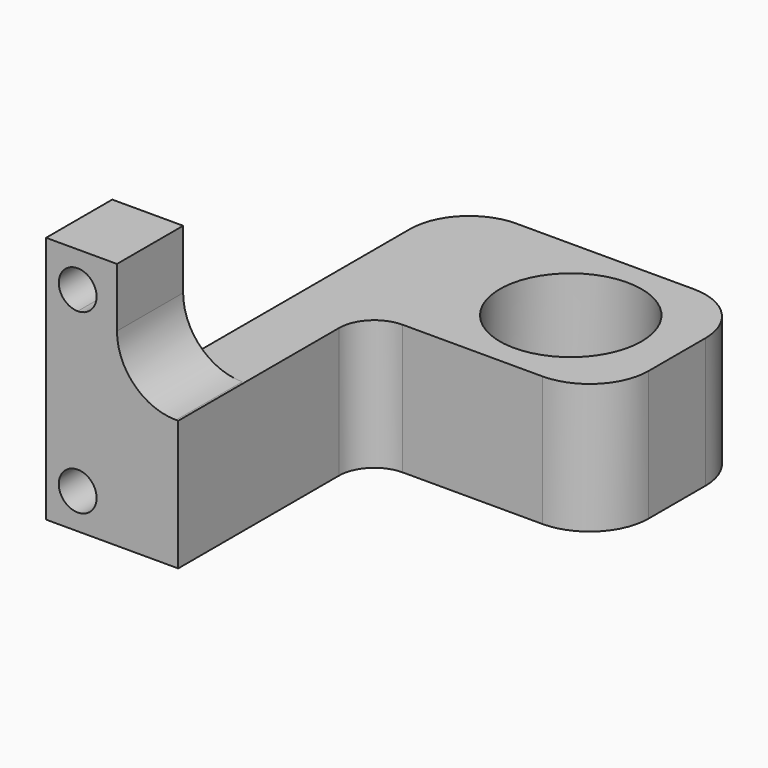
from build123d import *

# Parameters (mm, degrees)
F0_W     = 31
F0_H     = 36
F1_DEPTH = 4
F2_R     = 6
F2_W     = 6
F2_H     = 29
F2_W_2   = 19.817460835
F2_H_2   = 20
F3_DEPTH = 25
F4_W     = 6
F4_H     = 7
F4_R     = 6
F5_DEPTH = 7
F6_DEPTH = 17
F8_DEPTH = 25
F9_F1_R  = 5
F9_F2_R  = 5
F10_R    = 3


# Not quite as in the source:
# - two fillets or chamfers of one size are made in one step


with BuildPart() as f1:
    # F0 (on Top) → F1 (new body)
    with BuildSketch(Plane.XY):
        with Locations((15.5, 18)):
            Rectangle(F0_W, F0_H)
    extrude(amount=F1_DEPTH)

    # F2 (on face) → F3 (cut)
    with BuildSketch(Plane.XY.offset(4)):
        with Locations((22, 28)):
            Circle(F2_R)
        with Locations((3, 21.5)):
            Rectangle(F2_W, F2_H)
        with Locations((21.0912695825, 10)):
            Rectangle(F2_W_2, F2_H_2)
    extrude(amount=-F3_DEPTH, mode=Mode.SUBTRACT)

    # F4 (on face) → F5 (join)
    with BuildSketch(Plane.XY.offset(4)):
        with Locations((3, 3.5)):
            Rectangle(F4_W, F4_H)
        Polygon((6, 36), (6, 7), (6, 0), (11.182539165, 0), (11.182539165, 20), (31, 20), (31, 36), align=None)
        with Locations((22, 28)):
            Circle(F4_R, mode=Mode.SUBTRACT)
    extrude(amount=F5_DEPTH)

    # F4 (on face) → F6 (join)
    with BuildSketch(Plane.XY.offset(4)):
        with Locations((3, 3.5)):
            Rectangle(F4_W, F4_H)
    extrude(amount=F6_DEPTH)

    # F7 (on face) → F8 (cut)
    with BuildSketch(Plane.XZ):
        with BuildLine():
            ThreePointArc((4.275, 3), (3.8063708499, 4.1313708499), (2.675, 4.6))
            ThreePointArc((2.675, 4.6), (1.5436291501, 1.8686291501), (4.275, 3))
        make_face()
        with BuildLine():
            ThreePointArc((4.275, 18), (1.5436291501, 19.1313708499), (2.675, 16.4))
            ThreePointArc((2.675, 16.4), (3.8063708499, 16.8686291501), (4.275, 18))
        make_face()
    extrude(amount=-F8_DEPTH, mode=Mode.SUBTRACT)

    # F9: fillet of radius 5 on 4 edges, made by hand

    # F9_f1
    f9_f1_edges = [f1.edges().sort_by_distance(p)[0] for p in [
        (6, 3.5, 11),
    ]]
    fillet(f9_f1_edges, radius=F9_F1_R)

    # F9_f2
    f9_f2_edges = [f1.edges().sort_by_distance(p)[0] for p in [
        (31, 36, 5.5),
        (6, 36, 5.5),
        (31, 20, 5.5),
    ]]
    fillet(f9_f2_edges, radius=F9_F2_R)

    # F10
    f10_edges = [f1.edges().sort_by_distance(p)[0] for p in [
        (11.182539, 20, 5.5),
    ]]
    fillet(f10_edges, radius=F10_R)


solid = f1.part
